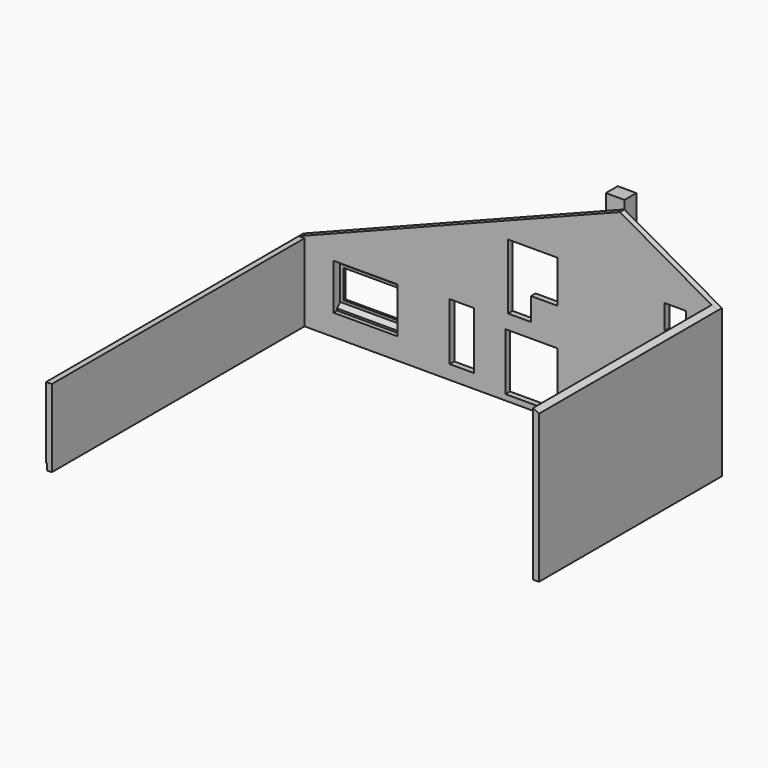
from build123d import *

# Parameters (mm, degrees)
F1_DEPTH      = 2224.5
F1_DEPTH_BACK = 490
F2_W          = 850.5
F2_H          = 2000.5
F2_W_2        = 1820
F2_W_3        = 1220
F2_H_2        = 1400
F3_DEPTH      = 200
F4_W          = 2240
F4_H          = 1600.5
F5_DEPTH      = 200
F7_DEPTH      = 2240
F9_DEPTH      = 80
F10_START     = -2320
F10_DEPTH     = 80
F11_W         = 2000.5
F11_H         = 1000.5
F12_DEPTH     = 80
F14_DEPTH     = 200
F14_FACE_W    = 200
F14_FACE_H    = 7800.5
F15_REACH     = 12195.4815488388
F2_W_4        = 750
F2_H_3        = 850
F16_DEPTH     = 200
F18_DEPTH     = 200
F20_DEPTH     = 520
F22_DEPTH     = 25
F23_W         = 11225.5
F23_H         = 220
F24_DEPTH     = 25
F25_R         = 20
F26_DEPTH     = 500


with BuildPart() as f1:
    # F0 (on Top) → F1 (new body, two sides)
    with BuildSketch(Plane.XY) as f1_sk:
        Polygon((8510, 0), (-6130, 0), (-6130, -11250.5), (-5930, -11250.5), (-5930, -200), (8310, -200), (8310, -8000.5), (8510, -8000.5), align=None)
    extrude(amount=F1_DEPTH)
    extrude(f1_sk.sketch, amount=-F1_DEPTH_BACK)

    # F2 (on face) → F3 (cut, through all)
    with BuildSketch(Plane(origin=(0, 0, 0), x_dir=(-1, 0, 0), z_dir=(0, 1, 0))):
        with Locations((425.25, 1000.25)):
            Rectangle(F2_W, F2_H)
        with Locations((-2010, 710.25)):
            Rectangle(F2_W_2, F2_H)
        with Locations((-7140, 1060)):
            Rectangle(F2_W_3, F2_H_2)
    extrude(amount=-F3_DEPTH, mode=Mode.SUBTRACT)

    # F4 (on face) → F5 (cut, through all)
    with BuildSketch(Plane(origin=(0, 0, 0), x_dir=(-1, 0, 0), z_dir=(0, 1, 0))):
        with Locations((3800, 1060.75)):
            Rectangle(F4_W, F4_H)
    extrude(amount=-F5_DEPTH, mode=Mode.SUBTRACT)

    # F6 (on face) → F7 (join, through all)
    with BuildSketch(Plane(origin=(-2680, 0, 0), x_dir=(0, -1, 0), z_dir=(-1, 0, 0))):
        Polygon((44.6384282427, 1861), (0, 1861), (-175, 1683.25), (-175, 438.25), (0, 260.5), (44.6384282427, 260.5), (44.6384282427, 329.1895949349), (-95, 471.0223413358), (-95, 1650.4776586642), (44.6384282427, 1792.310405065), align=None)
    extrude(amount=F7_DEPTH)

    # F8 (on face) → F9 (join)
    with BuildSketch(Plane.YZ.offset(-2680)):
        Polygon((175, 438.25), (175, 1683.25), (0, 1861), (0, 260.5), align=None)
    extrude(amount=F9_DEPTH)

    # F9_face (on face) → F10 (join)
    with BuildSketch(Plane(origin=(-2600, 83.8560885609, 1060.75), x_dir=(0, 1, 0), z_dir=(1, 0, 0)).offset(F10_START)):
        Polygon((91.1439114391, -622.5), (91.1439114391, 622.5), (-83.8560885609, 800.25), (-83.8560885609, -800.25), align=None)
    extrude(amount=-F10_DEPTH)

    # F11 (on face) → F12 (cut, through all)
    with BuildSketch(Plane(origin=(0, 175, 0), x_dir=(-1, 0, 0), z_dir=(0, 1, 0))):
        with Locations((3800, 1060.7499999998)):
            Rectangle(F11_W, F11_H)
    extrude(amount=-F12_DEPTH, mode=Mode.SUBTRACT)

    # F13 (on face) → F14 (join, through all)
    with BuildSketch(Plane(origin=(0, 0, 0), x_dir=(-1, 0, 0), z_dir=(0, 1, 0))):
        Polygon((6130, 2224.5), (-5100.5, 6616.9170318604), (-8510, 4687.5), (-8510, 2224.5), align=None)
    extrude(amount=-F14_DEPTH)

    f15_end = Plane(origin=(6805.25, -100, 5652.2085159302), x_dir=(0.870310319, 0, -0.4925037549), z_dir=(0.4925037549, 0, 0.870310319))
    # F14_face (on face) → F15 (join, up to a plane its end follows)
    with BuildSketch(Plane(origin=(8410, -4100.25, 2224.5), x_dir=(1, 0, 0), z_dir=(0, 0, 1))):
        Rectangle(F14_FACE_W, F14_FACE_H)
    f15_long = extrude(amount=F15_REACH, mode=Mode.PRIVATE)
    add(split(f15_long, bisect_by=f15_end, keep=Keep.BOTTOM, mode=Mode.PRIVATE))

    # F2 (on face) → F16 (cut, through all)
    with BuildSketch(Plane(origin=(0, 0, 0), x_dir=(-1, 0, 0), z_dir=(0, 1, 0))):
        with Locations((-7044.5, 3900.5)):
            Rectangle(F2_W_4, F2_H_3)
    extrude(amount=-F16_DEPTH, mode=Mode.SUBTRACT)

    # F17 (on face) → F18 (cut, through all)
    with BuildSketch(Plane(origin=(0, 0, 0), x_dir=(-1, 0, 0), z_dir=(0, 1, 0))):
        Polygon((-2920, 4501), (-2920, 3020.5), (-1990, 3020.5), (-1990, 2220.5), (-1189.5, 2220.5), (-1189.5, 4501), align=None)
    extrude(amount=-F18_DEPTH, mode=Mode.SUBTRACT)

    # F19 (on face) → F20 (join)
    with BuildSketch(Plane(origin=(0, 0, 0), x_dir=(-1, 0, 0), z_dir=(0, 1, 0))):
        Polygon((-4450, 6910.5), (-5100.5, 6910.5), (-5100.5, 1839.3845928857), (-5770, 1270.3168166825), (-5770, -490), (-4450, -490), align=None)
    extrude(amount=F20_DEPTH)

    # F21 (on face) → F22 (cut)
    with BuildSketch(Plane(origin=(0, 0, 0), x_dir=(-1, 0, 0), z_dir=(0, 1, 0))):
        Polygon((6130, -490), (6130, -270), (-90, -270), (-90, -450), (-4450, -450), (-4450, -490), align=None)
    extrude(amount=-F22_DEPTH, mode=Mode.SUBTRACT)

    # F23 (on face) → F24 (cut)
    with BuildSketch(Plane(origin=(-6130, 0, 0), x_dir=(0, -1, 0), z_dir=(-1, 0, 0))):
        with Locations((5637.75, -380)):
            Rectangle(F23_W, F23_H)
    extrude(amount=-F24_DEPTH, mode=Mode.SUBTRACT)


with BuildPart() as f26:
    # F25 (on face) → F26 (new body)
    with BuildSketch(Plane(origin=(0, 0, -490), x_dir=(1, 0, 0), z_dir=(0, 0, -1))):
        with Locations((-6070, -190)):
            Circle(F25_R)
    extrude(amount=-F26_DEPTH)


with BuildPart() as f26b:
    # F25 (on face) → F26, piece 2 (new body)
    with BuildSketch(Plane(origin=(0, 0, -490), x_dir=(1, 0, 0), z_dir=(0, 0, -1))):
        with Locations((-6070, -90)):
            Circle(F25_R)
    extrude(amount=-F26_DEPTH)


with BuildPart() as f26c:
    # F25 (on face) → F26, piece 3 (new body)
    with BuildSketch(Plane(origin=(0, 0, -490), x_dir=(1, 0, 0), z_dir=(0, 0, -1))):
        with Locations((-6260, 70)):
            Circle(F25_R)
    extrude(amount=-F26_DEPTH)


with BuildPart() as f26d:
    # F25 (on face) → F26, piece 4 (new body)
    with BuildSketch(Plane(origin=(0, 0, -490), x_dir=(1, 0, 0), z_dir=(0, 0, -1))):
        with Locations((-6260, 240)):
            Circle(F25_R)
    extrude(amount=-F26_DEPTH)


with BuildPart() as f26e:
    # F25 (on face) → F26, piece 5 (new body)
    with BuildSketch(Plane(origin=(0, 0, -490), x_dir=(1, 0, 0), z_dir=(0, 0, -1))):
        with Locations((-6360, 240)):
            Circle(F25_R)
    extrude(amount=-F26_DEPTH)


with BuildPart() as f26f:
    # F25 (on face) → F26, piece 6 (new body)
    with BuildSketch(Plane(origin=(0, 0, -490), x_dir=(1, 0, 0), z_dir=(0, 0, -1))):
        with Locations((-6360, 70)):
            Circle(F25_R)
    extrude(amount=-F26_DEPTH)


solid = Compound([f1.part, f26.part, f26b.part, f26c.part, f26d.part, f26e.part, f26f.part])
